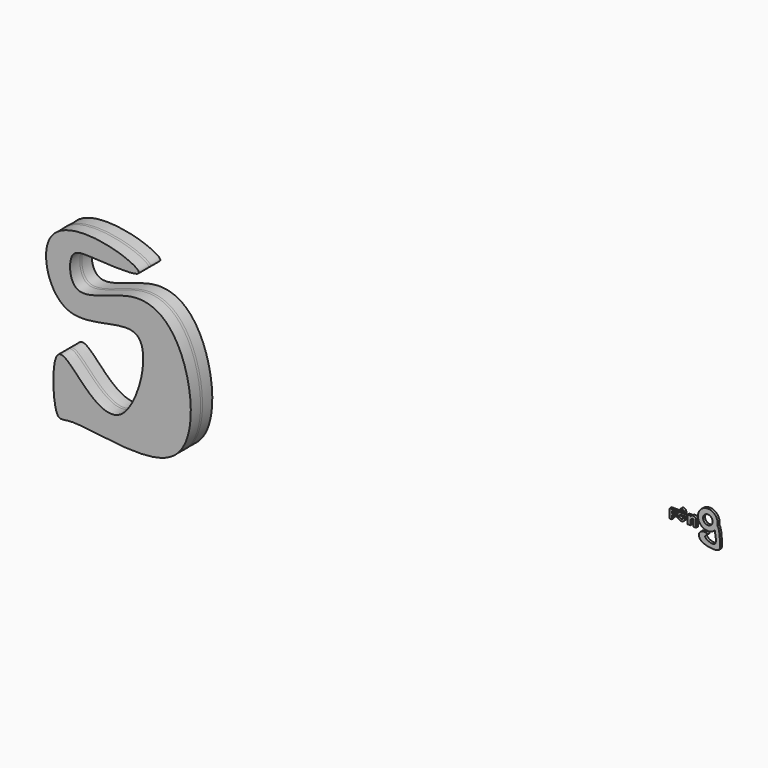
from build123d import *

# Parameters (mm, degrees)
F1_DEPTH  = 25.4
F2_R      = 20.1515683271
F3_DEPTH  = 25.4
F5_DEPTH  = 25.4
F6_R      = 49.5474241776
F7_DEPTH  = 25.4
F9_DEPTH  = 25.4
F10_DEPTH = 127
F11_DEPTH = 127


with BuildPart() as f1:
    # F0 (on Front) → F1 (new body)
    with BuildSketch(Plane.XZ):
        Polygon((4.896000959, 60.6670416892), (-50.7932938635, 60.6670416892), (-72.532787919, 60.6670416892), (-72.532787919, -33.2959592342), (-50.7932938635, -33.2959592342), (-50.7932938635, 6.2463153154), (0, 6.2463153154), (0, 22.8114202619), (-50.7932938635, 22.8114202619), (-50.7932938635, 44.4013550878), (4.896000959, 44.4013550878), align=None)
    extrude(amount=F1_DEPTH)


with BuildPart() as f3:
    # F2 (on Front) → F3 (new body)
    with BuildSketch(Plane.XZ):
        with BuildLine():
            Line((69.2080184817, 71.8808546662), (69.2080184817, 57.0950497716))
            ThreePointArc((69.2080184817, 57.0950497716), (20.9506599051, -7.0739813824), (80.7534490159, 46.4989934334))
            Line((80.7534490159, 46.4989934334), (78.764423728, 79.1520401835))
            ThreePointArc((78.764423728, 79.1520401835), (54.4474535963, 96.4283882368), (28.9048738778, 81.0217708349))
            Line((28.9048738778, 81.0217708349), (39.9155244231, 74.5815783739))
            ThreePointArc((39.9155244231, 74.5815783739), (55.5125178382, 83.5431683785), (69.2080184817, 71.8808546662))
        make_face()
        with Locations((48.2254512608, 22.6445477456)):
            Circle(F2_R, mode=Mode.SUBTRACT)
    extrude(amount=F3_DEPTH)


with BuildPart() as f5:
    # F4 (on Front) → F5 (new body)
    with BuildSketch(Plane.XZ):
        with BuildLine():
            Line((143.564581871, 63.1934255362), (111.563526094, 63.1934255362))
            Line((111.563526094, 63.1934255362), (111.563526094, -25.4951938987))
            Line((111.563526094, -25.4951938987), (143.564581871, -25.4951938987))
            Line((143.564581871, -25.4951938987), (143.564581871, 18.8491158187))
            ThreePointArc((143.564581871, 18.8491158187), (154.4043540585, 37.3283583229), (175.1084774733, 42.834930599))
            Line((175.1084774733, 42.834930599), (175.1084774733, -28.2381400466))
            Line((175.1084774733, -28.2381400466), (202.5379389524, -28.2381400466))
            Line((202.5379389524, -28.2381400466), (202.5379389524, 53.5931102931))
            ThreePointArc((202.5379389524, 53.5931102931), (173.4391114232, 70.9564445373), (143.564581871, 54.9645833671))
            Line((143.564581871, 54.9645833671), (143.564581871, 63.1934255362))
        make_face()
    extrude(amount=F5_DEPTH)


with BuildPart() as f7:
    # F6 (on Front) → F7 (new body)
    with BuildSketch(Plane.XZ):
        with BuildLine():
            add(Edge.make_bspline(
                [(423.6851538527, 62.3972549785), (415.2890698824, 72.249644405), (388.7027752218, 70.9058885795), (390.3335545605, 40.2469822597), (395.5211865422, 11.3402300988)],
                knots=[0.863337876, 0.863337876, 0.863337876, 0.863337876, 0.9187549499, 1, 1, 1, 1], degree=3))
            ThreePointArc((423.6851538527, 62.3972549785), (233.8136390734, 133.8373892581), (395.5211865422, 11.3402300988))
        make_face()
        with Locations((323.5620558262, 84.3305587769)):
            Circle(F6_R, mode=Mode.SUBTRACT)
        with BuildLine():
            add(Edge.make_bspline(
                [(395.5211865422, 11.3402300988), (403.3968523027, -32.5449026633), (436.7683420202, -162.4469960687), (253.4268012825, -79.0209266907), (355.534441953, -45.0547650507), (231.2767549114, -24.4184514926), (216.6868917952, -153.8545946428), (442.8536893784, -179.6889597751), (454.4604391253, -115.1261400281), (445.6974879499, 36.5668692321), (423.6851538527, 62.3972549785)],
                knots=[0, 0, 0, 0, 0.123343148, 0.2339023765, 0.3021466231, 0.3926117963, 0.4886692082, 0.6368200822, 0.7180488163, 0.863337876, 0.863337876, 0.863337876, 0.863337876], degree=3))
            add(Edge.make_bspline(
                [(423.6851538527, 62.3972549785), (415.2890698824, 72.249644405), (388.7027752218, 70.9058885795), (390.3335545605, 40.2469822597), (395.5211865422, 11.3402300988)],
                knots=[0.863337876, 0.863337876, 0.863337876, 0.863337876, 0.9187549499, 1, 1, 1, 1], degree=3))
        make_face()
    extrude(amount=F7_DEPTH)


with BuildPart() as f9:
    # F8 (on Front) → F9 (new body)
    with BuildSketch(Plane.XZ):
        with BuildLine():
            add(Edge.make_bspline(
                [(-5789.8721694946, 646.7041969299), (-6029.0974564563, 702.5544866781), (-6600.2036870222, 692.4582475207), (-6330.9393082426, -365.6849305228), (-5247.260869054, 261.6542176688), (-5583.4771670994, -1053.983190959), (-6049.4082894386, -767.8965865714), (-6410.0912093828, -278.890270212), (-6380.6127365378, -1165.9084787937), (-6179.4191681434, -1017.7822785815), (-4856.7559437472, -1390.1476170648), (-4940.9912866156, -20.9547533999), (-5486.0163828131, 417.5691986973), (-6194.1273480798, -38.9251401465), (-6231.23958143, 501.8405446254), (-5981.5455739721, 488.8030796811), (-5291.4631694677, 448.3549468047), (-5617.1348275726, 606.3763924607), (-5789.8721694946, 646.7041969299)],
                knots=[0, 0, 0, 0, 0.0692552473, 0.1384817025, 0.2118471534, 0.2881456467, 0.3433136131, 0.3948388618, 0.4590934257, 0.4923882186, 0.5815276731, 0.6669410696, 0.7344456887, 0.8021293852, 0.8488514416, 0.8903688476, 0.9499928813, 1, 1, 1, 1], degree=3))
        make_face()
    extrude(amount=F9_DEPTH)

    # F10 (add): a face of the model
    f10_faces = [f9.faces().sort_by_distance(p)[0] for p in [
        (-6050.0786856326, -25.4, -1069.7615712913),
    ]]
    extrude(f10_faces, amount=F10_DEPTH)

    # F11 (add): a face of the model
    f11_faces = [f9.faces().sort_by_distance(p)[0] for p in [
        (-6050.0786856326, 0, -1069.7615712913),
    ]]
    extrude(f11_faces, amount=F11_DEPTH)


solid = Compound([f1.part, f3.part, f5.part, f7.part, f9.part])
